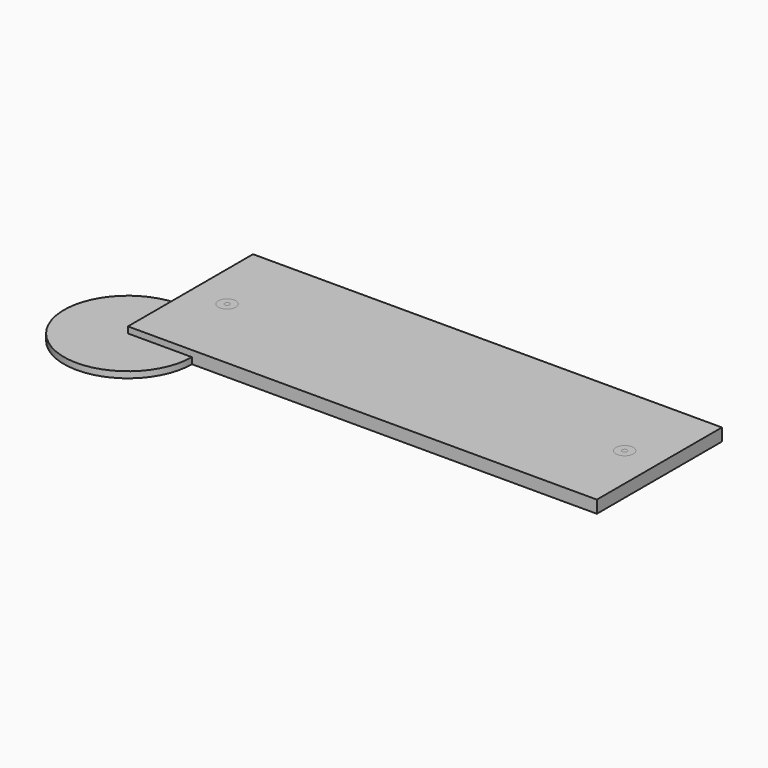
from build123d import *

# Parameters (mm, degrees)
F0_W     = 75
F0_H     = 25
F4_DEPTH = 0.4
F3_W     = 75
F3_H     = 25
F3_R     = 10.25
F5_DEPTH = 1.6
F2_W     = 75
F2_H     = 25
F6_DEPTH = 2
F1_R     = 1.4
F1_R_2   = 0.4
F7_DEPTH = 2
F8_R     = 10.225
F9_DEPTH = 1


with BuildPart() as f4:
    # F0 (on Top) → F4 (new body)
    with BuildSketch(Plane.XY):
        with Locations((37.5, 12.5)):
            Rectangle(F0_W, F0_H)
    extrude(amount=F4_DEPTH)

    # F3 (on Top) → F5 (join)
    with BuildSketch(Plane.XY):
        with Locations((37.5, 12.5)):
            Rectangle(F3_W, F3_H)
        with Locations((41.7743064463, 12.5000113621)):
            Circle(F3_R, mode=Mode.SUBTRACT)
    extrude(amount=F5_DEPTH)

    # F2 (on Top) → F6 (join)
    with BuildSketch(Plane.XY):
        with Locations((37.5, 12.5)):
            Rectangle(F2_W, F2_H)
        with BuildLine():
            Line((20.9633884676, 8.163), (20.9633884676, 9.0255))
            ThreePointArc((20.9633884676, 9.0255), (21.0805457551, 9.3083427125), (21.3633884676, 9.4255))
            Line((21.3633884676, 9.4255), (24.7770920396, 9.4255))
            Line((24.7770920396, 9.4255), (32.905688939, 7.3625277004))
            Line((32.905688939, 7.3625277004), (24.7770920396, 5.3))
            Line((24.7770920396, 5.3), (21.3633884676, 5.3))
            ThreePointArc((21.3633884676, 5.3), (21.0805457551, 5.4171572875), (20.9633884676, 5.7))
            Line((20.9633884676, 5.7), (20.9633884676, 6.563))
            ThreePointArc((20.9633884676, 6.563), (20.6146360295, 7.0607260803), (20.0873884676, 7.363))
            ThreePointArc((20.0873884676, 7.363), (20.6146360295, 7.6652739197), (20.9633884676, 8.163))
        make_face(mode=Mode.SUBTRACT)
        with BuildLine():
            ThreePointArc((17.3638739623, 7.863), (17.0810312498, 7.9801572875), (16.9638739623, 8.263))
            Line((16.9638739623, 8.263), (16.9638739623, 11.5626839529))
            ThreePointArc((16.9638739623, 11.5626839529), (16.5400607006, 12.1874218401), (15.8528853208, 12.5))
            ThreePointArc((15.8528853208, 12.5), (16.6743001007, 13.0131119919), (16.9638739623, 13.9373160471))
            Line((16.9638739623, 13.9373160471), (16.9638739623, 16.7375))
            ThreePointArc((16.9638739623, 16.7375), (17.0810312498, 17.0203427125), (17.3638739623, 17.1375))
            Line((17.3638739623, 17.1375), (19.5638739623, 17.1375))
            ThreePointArc((19.5638739623, 17.1375), (19.8467166748, 17.0203427125), (19.9638739623, 16.7375))
            Line((19.9638739623, 16.7375), (19.9638739623, 15.5745))
            Line((19.9638739623, 15.5745), (19.9638739623, 15.0745))
            Line((19.9638739623, 15.0745), (19.9638739623, 14.9745))
            ThreePointArc((19.9638739623, 14.9745), (20.0810312498, 14.6916572875), (20.3638739623, 14.5745))
            Line((20.3638739623, 14.5745), (24.7770920396, 14.5745))
            Line((24.7770920396, 14.5745), (31.5258568066, 12.49955))
            Line((31.5258568066, 12.49955), (24.7770920396, 10.4255))
            Line((24.7770920396, 10.4255), (20.3633884676, 10.4255))
            ThreePointArc((20.3633884676, 10.4255), (20.0805457551, 10.3083427125), (19.9633884676, 10.0255))
            Line((19.9633884676, 10.0255), (19.9633884676, 9.9255))
            Line((19.9633884676, 9.9255), (19.9633884676, 9.4255))
            Line((19.9633884676, 9.4255), (19.9633884676, 8.263))
            ThreePointArc((19.9633884676, 8.263), (19.8462311801, 7.9801572875), (19.5633884676, 7.863))
            Line((19.5633884676, 7.863), (17.3638739623, 7.863))
        make_face(mode=Mode.SUBTRACT)
        with BuildLine():
            ThreePointArc((21.3638739623, 15.5745), (21.0810312498, 15.6916572875), (20.9638739623, 15.9745))
            Line((20.9638739623, 15.9745), (20.9638739623, 16.8364493074))
            ThreePointArc((20.9638739623, 16.8364493074), (20.61521579, 17.3303099873), (20.0904036045, 17.6303650859))
            ThreePointArc((20.0904036045, 17.6303650859), (20.61521579, 17.9304201845), (20.9638739623, 18.4242808644))
            Line((20.9638739623, 18.4242808644), (20.9638739623, 19.3))
            ThreePointArc((20.9638739623, 19.3), (21.0810312498, 19.5828427125), (21.3638739623, 19.7))
            Line((21.3638739623, 19.7), (24.7770920396, 19.7))
            Line((24.7770920396, 19.7), (32.9031571746, 17.6303650859))
            Line((32.9031571746, 17.6303650859), (24.7770920396, 15.5745))
            Line((24.7770920396, 15.5745), (21.3638739623, 15.5745))
        make_face(mode=Mode.SUBTRACT)
        with BuildLine():
            ThreePointArc((21.3633884676, 9.4255), (21.0805457551, 9.3083427125), (20.9633884676, 9.0255))
            Line((20.9633884676, 9.0255), (20.9633884676, 8.163))
            ThreePointArc((20.9633884676, 8.163), (20.6146360295, 7.6652739197), (20.0873884676, 7.363))
            ThreePointArc((20.0873884676, 7.363), (20.6146360295, 7.0607260803), (20.9633884676, 6.563))
            Line((20.9633884676, 6.563), (20.9633884676, 5.7))
            ThreePointArc((20.9633884676, 5.7), (21.0805457551, 5.4171572875), (21.3633884676, 5.3))
            Line((21.3633884676, 5.3), (24.7770920396, 5.3))
            Line((24.7770920396, 5.3), (32.905688939, 7.3625277004))
            Line((32.905688939, 7.3625277004), (24.7770920396, 9.4255))
            Line((24.7770920396, 9.4255), (21.3633884676, 9.4255))
        make_face()
        with BuildLine():
            Line((16.9638739623, 11.5626839529), (16.9638739623, 8.263))
            ThreePointArc((16.9638739623, 8.263), (17.0810312498, 7.9801572875), (17.3638739623, 7.863))
            Line((17.3638739623, 7.863), (19.5633884676, 7.863))
            ThreePointArc((19.5633884676, 7.863), (19.8462311801, 7.9801572875), (19.9633884676, 8.263))
            Line((19.9633884676, 8.263), (19.9633884676, 9.4255))
            Line((19.9633884676, 9.4255), (19.9633884676, 9.9255))
            Line((19.9633884676, 9.9255), (19.9633884676, 10.0255))
            ThreePointArc((19.9633884676, 10.0255), (20.0805457551, 10.3083427125), (20.3633884676, 10.4255))
            Line((20.3633884676, 10.4255), (24.7770920396, 10.4255))
            Line((24.7770920396, 10.4255), (31.5258568066, 12.49955))
            Line((31.5258568066, 12.49955), (24.7770920396, 14.5745))
            Line((24.7770920396, 14.5745), (20.3638739623, 14.5745))
            ThreePointArc((20.3638739623, 14.5745), (20.0810312498, 14.6916572875), (19.9638739623, 14.9745))
            Line((19.9638739623, 14.9745), (19.9638739623, 15.0745))
            Line((19.9638739623, 15.0745), (19.9638739623, 15.5745))
            Line((19.9638739623, 15.5745), (19.9638739623, 16.7375))
            ThreePointArc((19.9638739623, 16.7375), (19.8467166748, 17.0203427125), (19.5638739623, 17.1375))
            Line((19.5638739623, 17.1375), (17.3638739623, 17.1375))
            ThreePointArc((17.3638739623, 17.1375), (17.0810312498, 17.0203427125), (16.9638739623, 16.7375))
            Line((16.9638739623, 16.7375), (16.9638739623, 13.9373160471))
            ThreePointArc((16.9638739623, 13.9373160471), (16.6743001007, 13.0131119919), (15.8528853208, 12.5))
            ThreePointArc((15.8528853208, 12.5), (16.5400607006, 12.1874218401), (16.9638739623, 11.5626839529))
        make_face()
        with BuildLine():
            Line((20.9638739623, 16.8364493074), (20.9638739623, 15.9745))
            ThreePointArc((20.9638739623, 15.9745), (21.0810312498, 15.6916572875), (21.3638739623, 15.5745))
            Line((21.3638739623, 15.5745), (24.7770920396, 15.5745))
            Line((24.7770920396, 15.5745), (32.9031571746, 17.6303650859))
            Line((32.9031571746, 17.6303650859), (24.7770920396, 19.7))
            Line((24.7770920396, 19.7), (21.3638739623, 19.7))
            ThreePointArc((21.3638739623, 19.7), (21.0810312498, 19.5828427125), (20.9638739623, 19.3))
            Line((20.9638739623, 19.3), (20.9638739623, 18.4242808644))
            ThreePointArc((20.9638739623, 18.4242808644), (20.61521579, 17.9304201845), (20.0904036045, 17.6303650859))
            ThreePointArc((20.0904036045, 17.6303650859), (20.61521579, 17.3303099873), (20.9638739623, 16.8364493074))
        make_face()
    extrude(amount=F6_DEPTH)


with BuildPart() as f7:
    # F1 (on Top) → F7 (new body)
    with BuildSketch(Plane.XY):
        with Locations((5.882635247, 12.4678043649)):
            Circle(F1_R)
        with Locations((5.882635247, 12.4678043649)):
            Circle(F1_R_2, mode=Mode.SUBTRACT)
    extrude(amount=F7_DEPTH)


with BuildPart() as f7b:
    # F1 (on Top) → F7, piece 2 (new body)
    with BuildSketch(Plane.XY):
        with Locations((69.4437474012, 12.5000113621)):
            Circle(F1_R)
        with Locations((69.4437474012, 12.5000113621)):
            Circle(F1_R_2, mode=Mode.SUBTRACT)
    extrude(amount=F7_DEPTH)


with BuildPart() as f9:
    # F8 (on Top) → F9 (new body)
    with BuildSketch(Plane.XY):
        Circle(F8_R)
    extrude(amount=F9_DEPTH)


solid = Compound([f4.part, f7.part, f7b.part, f9.part])
